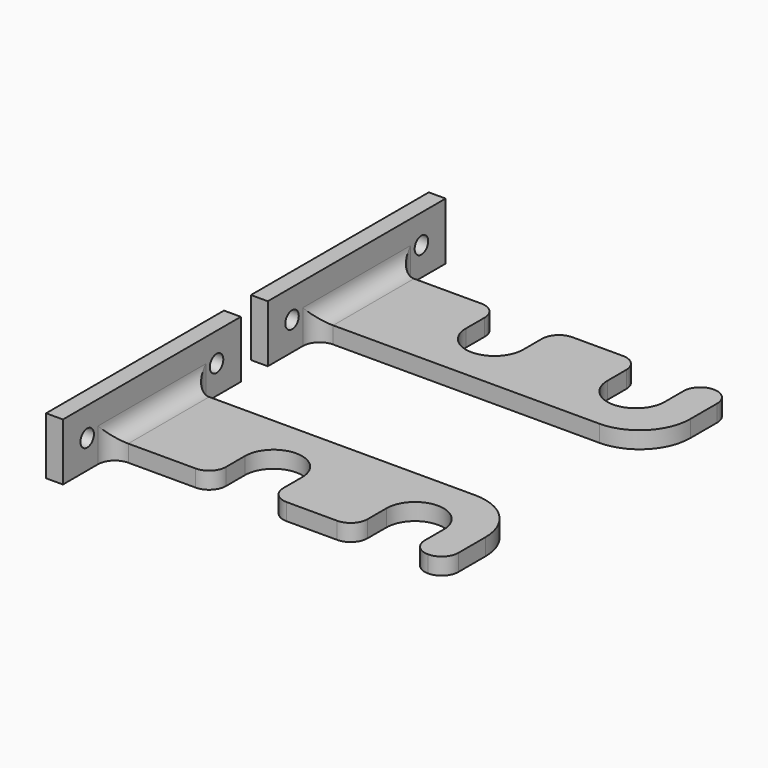
from build123d import *

# Parameters (mm, degrees)
F1_DEPTH = 5
F3_DEPTH = 12
F4_R     = 2.5
F5_DEPTH = 5.001
F6_R     = 4.99999
F7_R     = 15
F8_ANGLE = -90


# Not quite as in the source:
# - a fillet or chamfer is up to 0.001 mm smaller than in the source, because OpenCascade refuses the exact size


with BuildPart() as f1:
    # F0 (on Front) → F1 (new body)
    with BuildSketch(Plane.XZ):
        with BuildLine():
            ThreePointArc((45.2828197777, 12.5004108995), (36.7828197777, 4.0004108995), (28.2828197777, 12.5004108995))
            Line((28.2828197777, 12.5004108995), (28.2828197777, 24.5004108995))
            Line((28.2828197777, 24.5004108995), (-1.7171802223, 24.5004108995))
            Line((-1.7171802223, 24.5004108995), (-1.7171802223, -5.4995891005))
            Line((-1.7171802223, -5.4995891005), (97.2828197777, -5.4995891005))
            Line((97.2828197777, -5.4995891005), (97.2828197777, 12.5004108995))
            Line((97.2828197777, 12.5004108995), (97.2828197777, 24.5004108995))
            Line((97.2828197777, 24.5004108995), (87.2828197777, 24.5004108995))
            Line((87.2828197777, 24.5004108995), (87.2828197777, 12.5004108995))
            ThreePointArc((87.2828197777, 12.5004108995), (78.7828197777, 4.0004108995), (70.2828197777, 12.5004108995))
            Line((70.2828197777, 12.5004108995), (70.2828197777, 24.5004108995))
            Line((70.2828197777, 24.5004108995), (45.2828197777, 24.5004108995))
            Line((45.2828197777, 24.5004108995), (45.2828197777, 12.5004108995))
        make_face()
        Polygon((-1.7171802223, -5.4995891005), (-1.7171802223, 24.5004108995), (-1.7171802223, 42.5004108995), (-6.7171802223, 42.5004108995), (-6.7171802223, 24.5004108995), (-6.7171802223, 12.5004108995), (-6.7171802223, -5.4995891005), (-6.7171802223, -23.4995891005), (-1.7171802223, -23.4995891005), align=None)
    extrude(amount=F1_DEPTH)

    # F2 (on face) → F3 (join)
    with BuildSketch(Plane(origin=(0, 0, 0), x_dir=(-1, 0, 0), z_dir=(0, 1, 0))):
        Polygon((6.7171802223, 42.5004108995), (1.7171802223, 42.5004108995), (1.7171802223, 24.5004108995), (1.7171802223, -5.4995891005), (1.7171802223, -23.4255902469), (1.7171802223, -23.4995891005), (6.7171802223, -23.4995891005), align=None)
    extrude(amount=F3_DEPTH)

    # F4 (on face) → F5 (cut, through all)
    with BuildSketch(Plane.YZ.offset(-1.7171802223)):
        with Locations((3.5, 33.5004108995)):
            Circle(F4_R)
        with Locations((3.5, -14.4995891005)):
            Circle(F4_R)
    extrude(amount=-F5_DEPTH, mode=Mode.SUBTRACT)

    # F6 (radius 5 in the source; OpenCascade refuses exactly that, so slightly less here)
    f6_edges = [f1.edges().sort_by_distance(p)[0] for p in [
        (-1.71718, -2.5, 24.500411),
        (-1.71718, -2.5, -5.499589),
        (97.28282, -2.5, 24.500411),
        (28.28282, -2.5, 24.500411),
        (70.28282, -2.5, 24.500411),
        (87.28282, -2.5, 24.500411),
        (45.28282, -2.5, 24.500411),
        (-1.71718, 0, 9.500411),
    ]]
    fillet(f6_edges, radius=F6_R)

    # F7
    f7_edges = [f1.edges().sort_by_distance(p)[0] for p in [
        (97.28282, -2.5, -5.499589),
    ]]
    fillet(f7_edges, radius=F7_R)


with BuildPart() as f1_1:
    # F8: moved
    add(f1.part.rotate(Axis((42.7828147777, -5, -5.4995891005), (-1, 0, 0)), F8_ANGLE))


with BuildPart() as f10_1:
    # F10: instance of F1
    add(f1_1.part.mirror(Plane(origin=(-4.2171802223, 18, 3.0004108995), x_dir=(-1, 0, 0), z_dir=(0, 1, 0))))


solid = Compound([f1_1.part, f10_1.part])
